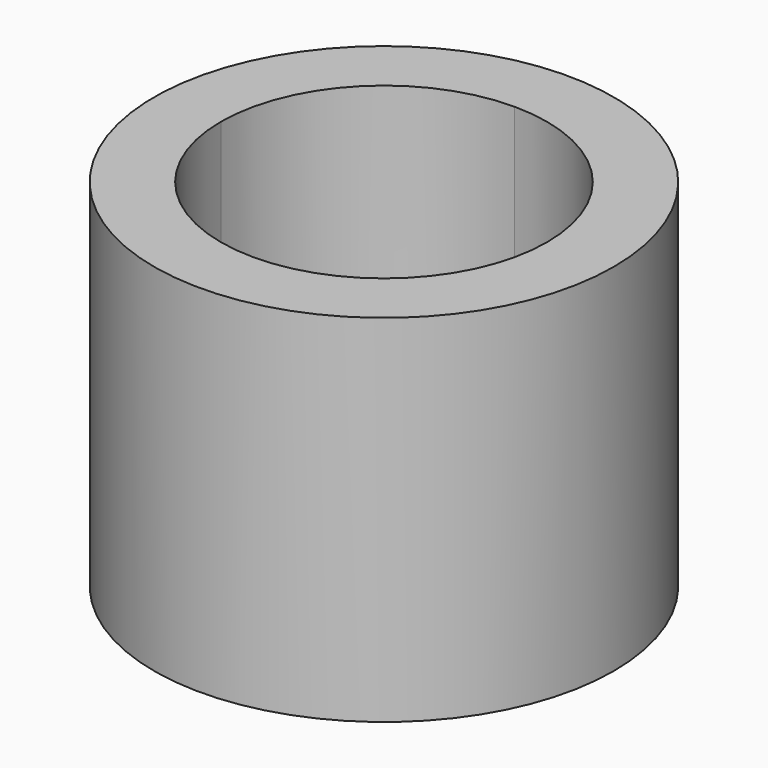
from build123d import *

# Parameters (mm, degrees)
F0_R     = 15.5
F1_DEPTH = 24


with BuildPart() as f1:
    # F0 (on Top) → F1 (new body)
    with BuildSketch(Plane.XY):
        Circle(F0_R)
        with BuildLine():
            ThreePointArc((0, 11.75), (8.3085046789, 8.3085046789), (11.75, 0))
            ThreePointArc((11.75, 0), (8.3085046789, -8.3085046789), (0, -11.75))
            ThreePointArc((0, -11.75), (-8.3085046789, -8.3085046789), (-11.75, 0))
            ThreePointArc((-11.75, 0), (-8.3085046789, 8.3085046789), (0, 11.75))
        make_face(mode=Mode.SUBTRACT)
        with BuildLine():
            ThreePointArc((0, 11), (7.7781745931, 7.7781745931), (11, 0))
            Line((11, 0), (11.75, 0))
            ThreePointArc((11.75, 0), (8.3085046789, 8.3085046789), (0, 11.75))
            Line((0, 11.75), (0, 11))
        make_face()
        with BuildLine():
            ThreePointArc((-11, 0), (-7.7781745931, 7.7781745931), (0, 11))
            Line((0, 11), (0, 11.75))
            ThreePointArc((0, 11.75), (-8.3085046789, 8.3085046789), (-11.75, 0))
            Line((-11.75, 0), (-11, 0))
        make_face()
        with BuildLine():
            Line((0, -11.75), (0, -11))
            ThreePointArc((0, -11), (-7.7781745931, -7.7781745931), (-11, 0))
            Line((-11, 0), (-11.75, 0))
            ThreePointArc((-11.75, 0), (-8.3085046789, -8.3085046789), (0, -11.75))
        make_face()
        with BuildLine():
            Line((11.75, 0), (11, 0))
            ThreePointArc((11, 0), (7.7781745931, -7.7781745931), (0, -11))
            Line((0, -11), (0, -11.75))
            ThreePointArc((0, -11.75), (8.3085046789, -8.3085046789), (11.75, 0))
        make_face()
    extrude(amount=F1_DEPTH)


solid = f1.part
